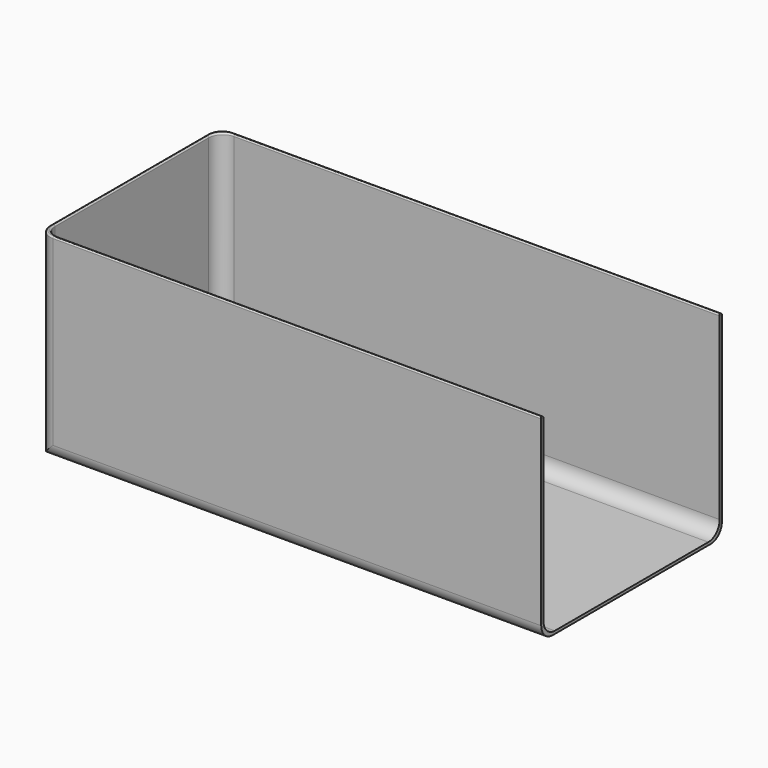
from build123d import *

# Parameters (mm, degrees)
F0_W     = 178
F0_H     = 80
F1_DEPTH = 70
F3_DEPTH = 69
F4_R     = 5
F5_R     = 0.49999


# Not quite as in the source:
# - a fillet or chamfer is up to 0.001 mm smaller than in the source, because OpenCascade refuses the exact size


with BuildPart() as f1:
    # F0 (on Top) → F1 (new body)
    with BuildSketch(Plane.XY):
        Rectangle(F0_W, F0_H)
    extrude(amount=F1_DEPTH)

    # F2 (on face) → F3 (cut)
    with BuildSketch(Plane.XY.offset(70)):
        Polygon((-88, -24.0239519626), (-88, -39), (-83.0030292273, -39), (89, -39), (89, 39), (-88, 39), align=None)
    extrude(amount=-F3_DEPTH, mode=Mode.SUBTRACT)

    # F4
    f4_edges = [f1.edges().sort_by_distance(p)[0] for p in [
        (-88, 39, 35.5),
        (0.5, 39, 1),
        (-88, 0, 1),
        (-88, -39, 35.5),
        (0.5, -39, 1),
        (0, 40, 0),
        (-89, 40, 35),
        (-89, -40, 35),
        (0, -40, 0),
    ]]
    fillet(f4_edges, radius=F4_R)

    # F5 (radius 0.5 in the source; OpenCascade refuses exactly that, so slightly less here)
    f5_edges = [f1.edges().sort_by_distance(p)[0] for p in [
        (-89, 0, 70),
        (-87.535534, 38.535534, 70),
        (-87.535534, -38.535534, 70),
        (2.5, 40, 70),
        (2.5, -40, 70),
        (89, 39.5, 70),
        (89, -39.5, 70),
        (3, 39, 70),
        (3, -39, 70),
        (-86.535534, 37.535534, 70),
        (-86.535534, -37.535534, 70),
        (-88, 0, 70),
    ]]
    fillet(f5_edges, radius=F5_R)


solid = f1.part
